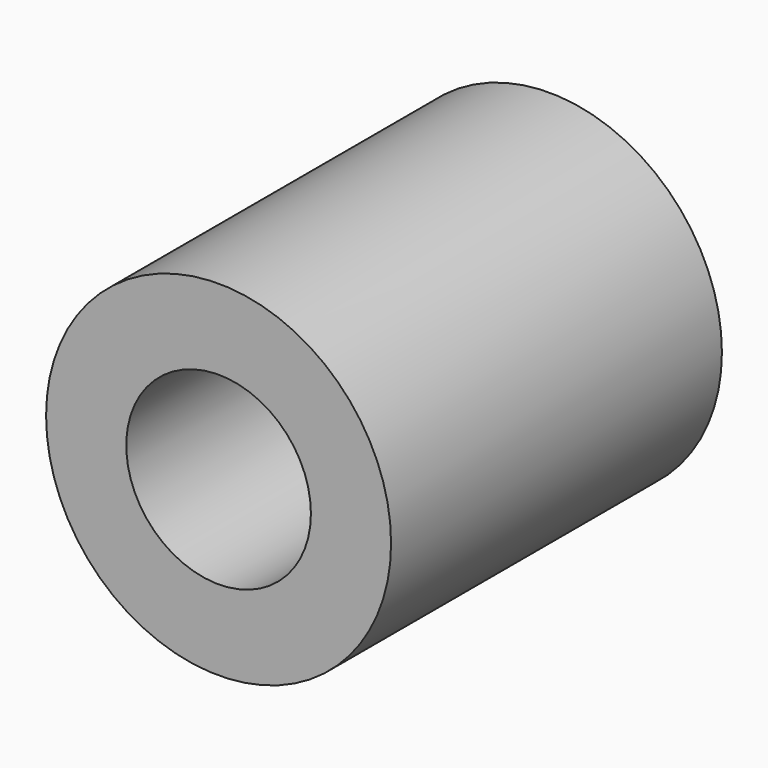
from build123d import *

# Parameters (mm, degrees)
F0_R     = 10.5945643577
F0_R_2   = 5.6705080361
F2_DEPTH = 25.4


# Not quite as in the source:
# - the program builds the solid bodies; features that only make, move or delete a surface that nothing else refers to are left out


with BuildPart() as f2:
    # F0 (on Front) → F2 (new body)
    with BuildSketch(Plane.XZ):
        Circle(F0_R)
        Circle(F0_R_2, mode=Mode.SUBTRACT)
    extrude(amount=F2_DEPTH)


solid = f2.part
